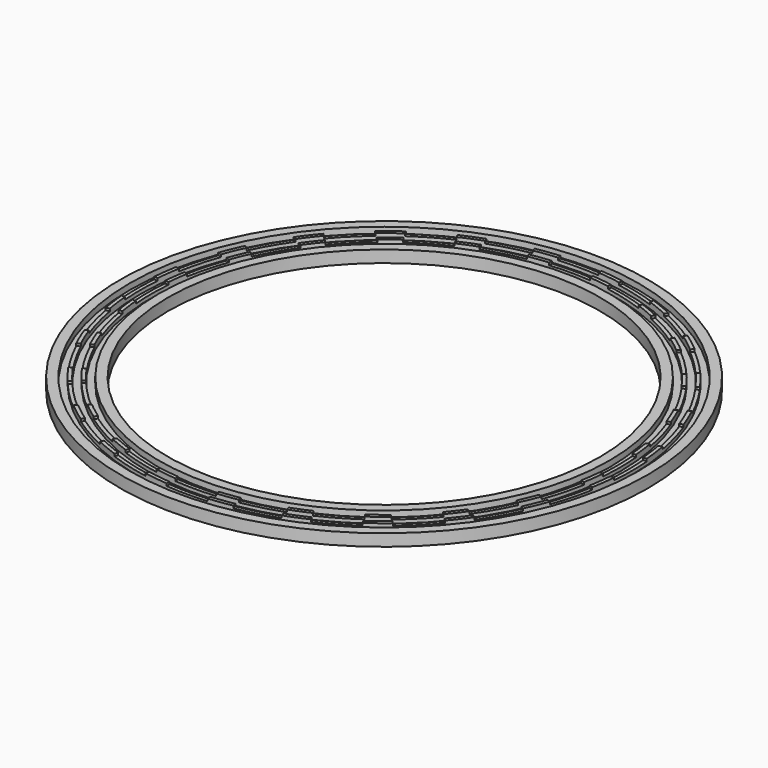
from build123d import *

# Parameters (mm, degrees)
F0_R            = 110
F0_R_2          = 90
F1_DEPTH        = 5
F2_W            = 17
F2_H            = 10
F4_DEPTH        = 1
F4_COPIES_COUNT = 24
F3_R            = 106
F3_R_2          = 103
F3_R_3          = 101.5
F3_R_4          = 98.5
F3_R_5          = 97
F3_R_6          = 94
F5_DEPTH        = 2.5


# Not quite as in the source:
# - a pattern or mirror of a feature is missing from the dataset's text; its kind, count and spacing are read off the source's solid


with BuildPart() as f1:
    # F0 (on Top) → F1 (new body)
    with BuildSketch(Plane.XY):
        Circle(F0_R)
        Circle(F0_R_2, mode=Mode.SUBTRACT)
    extrude(amount=F1_DEPTH)

    # F2 (on face) → F4 (cut)
    with BuildSketch(Plane.XY.offset(5)):
        with Locations((0, 100)):
            Rectangle(F2_W, F2_H)
    f4 = extrude(amount=-F4_DEPTH, mode=Mode.SUBTRACT)

    # F4_copies: F4 ×24 about axis
    f4_copies_axis = Axis((0, 0, 0), (0, 0, 1))
    for i in range(1, F4_COPIES_COUNT):
        add(f4.rotate(f4_copies_axis, i * 360 / F4_COPIES_COUNT), mode=Mode.SUBTRACT)

    # F3 (on face) → F5 (cut)
    with BuildSketch(Plane.XY.offset(5)):
        Circle(F3_R)
        Circle(F3_R_2, mode=Mode.SUBTRACT)
        Circle(F3_R_3)
        Circle(F3_R_4, mode=Mode.SUBTRACT)
        Circle(F3_R_5)
        Circle(F3_R_6, mode=Mode.SUBTRACT)
    extrude(amount=-F5_DEPTH, mode=Mode.SUBTRACT)


solid = f1.part
